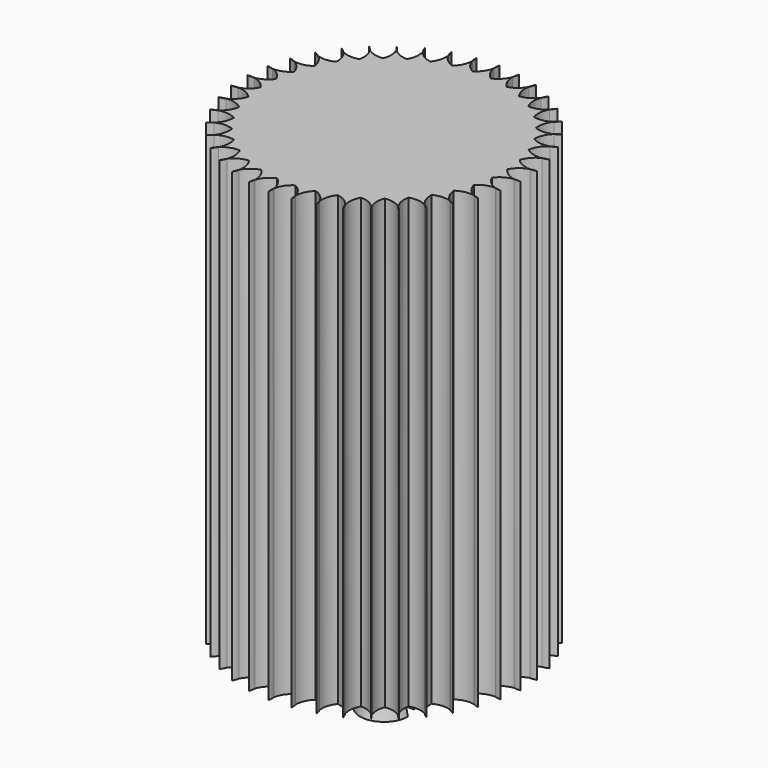
from build123d import *

# Parameters (mm, degrees)
F1_DEPTH  = 76.2
F2_R      = 43.4133239612
F3_DEPTH  = 101.6
F4_R      = 43.4133239612
F4_R_2    = 37.0604251076
F5_DEPTH  = 25.4
F5_TAPER  = -12
F6_W      = 117.5021827221
F6_H      = 89.2960429192
F7_DEPTH  = 25.4
F9_DEPTH  = 914.4
F11_R     = 53.1430060109
F11_R_2   = 54.2538976406
F12_DEPTH = 508


with BuildPart() as f1:
    # F0 (on Top) → F1 (new body)
    with BuildSketch(Plane.XY):
        with BuildLine():
            ThreePointArc((12.3147964478, 55.8442249894), (-0.0568873663, 74.6383593827), (-16.0615742207, 58.8229224086))
            Line((-16.0615742207, 58.8229224086), (-35.8245223761, 38.4155064821))
            Line((-35.8245223761, 38.4155064821), (-86.3886475563, 38.4155064821))
            Line((-86.3886475563, 38.4155064821), (-86.3886475563, -48.9976257086))
            Line((-86.3886475563, -48.9976257086), (99.40969944, -48.9976257086))
            Line((99.40969944, -48.9976257086), (101.6570031643, 38.4155064821))
            Line((101.6570031643, 38.4155064821), (32.9162478447, 38.4155064821))
            Line((32.9162478447, 38.4155064821), (12.3147964478, 55.8442249894))
        make_face()
    extrude(amount=F1_DEPTH)


with BuildPart() as f3:
    # F2 (on Top) → F3 (new body)
    with BuildSketch(Plane.XY):
        Circle(F2_R)
    extrude(amount=-F3_DEPTH)

    # F4 (on face) → F5 (join)
    with BuildSketch(Plane(origin=(0, 0, -101.6), x_dir=(1, 0, 0), z_dir=(0, 0, -1))):
        Circle(F4_R)
        Circle(F4_R_2, mode=Mode.SUBTRACT)
    extrude(amount=F5_DEPTH, taper=F5_TAPER)

    # F6 (on Front) → F7 (cut)
    with BuildSketch(Plane.XZ):
        with Locations((0, -93.4350788593)):
            Rectangle(F6_W, F6_H)
    extrude(amount=-F7_DEPTH, mode=Mode.SUBTRACT)


with BuildPart() as f9:
    # F8 (on Top) → F9 (new body)
    with BuildSketch(Plane.XY):
        with BuildLine():
            ThreePointArc((35.2223104144, -269.369402679), (35.5915835041, -275.9196411281), (36.9189268773, -282.3446038458))
            ThreePointArc((36.9189268773, -282.3446038458), (36.5496537876, -275.7943653967), (35.2223104144, -269.369402679))
        make_face()
    extrude(amount=F9_DEPTH)


with BuildPart() as f9b:
    # F8 (on Top) → F9, piece 2 (new body)
    with BuildSketch(Plane.XY):
        with BuildLine():
            ThreePointArc((-7.7040334356, -284.6438658243), (-7.0440771132, -278.1165046418), (-7.3499930812, -271.5630016263))
            ThreePointArc((-7.3499930812, -271.5630016263), (-8.0099494037, -278.0903628088), (-7.7040334356, -284.6438658243))
        make_face()
    extrude(amount=F9_DEPTH)


with BuildPart() as f9c:
    # F8 (on Top) → F9, piece 3 (new body)
    with BuildSketch(Plane.XY):
        with BuildLine():
            ThreePointArc((-52.1372948771, -279.9342511475), (-50.4643594574, -273.5904925269), (-49.7413153539, -267.0698182076))
            ThreePointArc((-49.7413153539, -267.0698182076), (-51.4142507736, -273.4135768282), (-52.1372948771, -279.9342511475))
        make_face()
    extrude(amount=F9_DEPTH)


with BuildPart() as f9d:
    # F8 (on Top) → F9, piece 4 (new body)
    with BuildSketch(Plane.XY):
        with BuildLine():
            ThreePointArc((-95.286763085, -268.3317261588), (-92.6420417903, -262.3277744912), (-90.9078413606, -256.0004895108))
            ThreePointArc((-90.9078413606, -256.0004895108), (-93.5525626554, -262.0044411784), (-95.286763085, -268.3317261588))
        make_face()
    extrude(amount=F9_DEPTH)


with BuildPart() as f9e:
    # F8 (on Top) → F9, piece 5 (new body)
    with BuildSketch(Plane.XY):
        with BuildLine():
            ThreePointArc((-136.0899549471, -250.1219835302), (-132.5385695929, -244.6056760315), (-129.8359146072, -238.6275791452))
            ThreePointArc((-129.8359146072, -238.6275791452), (-133.3872999614, -244.1438866439), (-136.0899549471, -250.1219835302))
        make_face()
    extrude(amount=F9_DEPTH)


with BuildPart() as f9f:
    # F8 (on Top) → F9, piece 6 (new body)
    with BuildSketch(Plane.XY):
        with BuildLine():
            ThreePointArc((-173.5421604617, -225.7534075598), (-169.1715579419, -220.8605740283), (-165.5669967354, -215.3788658216))
            ThreePointArc((-165.5669967354, -215.3788658216), (-169.9375992553, -220.2716993531), (-173.5421604617, -225.7534075598))
        make_face()
    extrude(amount=F9_DEPTH)


with BuildPart() as f9g:
    # F8 (on Top) → F9, piece 7 (new body)
    with BuildSketch(Plane.XY):
        with BuildLine():
            ThreePointArc((-206.7211820324, -195.8260334627), (-201.6389810861, -191.6771516982), (-197.2212699187, -186.82681002))
            ThreePointArc((-197.2212699187, -186.82681002), (-202.303470865, -190.9756917844), (-206.7211820324, -195.8260334627))
        make_face()
    extrude(amount=F9_DEPTH)


with BuildPart() as f9h:
    # F8 (on Top) → F9, piece 8 (new body)
    with BuildSketch(Plane.XY):
        with BuildLine():
            ThreePointArc((-234.8100420331, -161.0767725124), (-229.1413833145, -157.7740017534), (-224.0193008967, -153.674458113))
            ThreePointArc((-224.0193008967, -153.674458113), (-229.6879596153, -156.977228872), (-234.8100420331, -161.0767725124))
        make_face()
    extrude(amount=F9_DEPTH)


with BuildPart() as f9i:
    # F8 (on Top) → F9, piece 9 (new body)
    with BuildSketch(Plane.XY):
        with BuildLine():
            ThreePointArc((-257.1170995091, -122.3612668397), (-251.0015642092, -119.9859322634), (-245.3012332092, -116.738131031))
            ThreePointArc((-245.3012332092, -116.738131031), (-251.4167685092, -119.1134656072), (-257.1170995091, -122.3612668397))
        make_face()
    extrude(amount=F9_DEPTH)


with BuildPart() as f9j:
    # F8 (on Top) → F9, piece 10 (new body)
    with BuildSketch(Plane.XY):
        with BuildLine():
            ThreePointArc((-273.0930806725, -80.6328206836), (-266.6812535665, -79.2434109107), (-260.543035052, -76.9273237314))
            ThreePointArc((-260.543035052, -76.9273237314), (-266.954862158, -78.3167335043), (-273.0930806725, -80.6328206836))
        make_face()
    extrude(amount=F9_DEPTH)


with BuildPart() as f9k:
    # F8 (on Top) → F9, piece 11 (new body)
    with BuildSketch(Plane.XY):
        with BuildLine():
            ThreePointArc((-282.3446038458, -36.9189268773), (-275.7943653967, -36.5496537876), (-269.369402679, -35.2223104144))
            ThreePointArc((-269.369402679, -35.2223104144), (-275.9196411281, -35.5915835041), (-282.3446038458, -36.9189268773))
        make_face()
    extrude(amount=F9_DEPTH)


with BuildPart() as f9l:
    # F8 (on Top) → F9, piece 12 (new body)
    with BuildSketch(Plane.XY):
        with BuildLine():
            ThreePointArc((-284.6438658243, 7.7040334356), (-278.1165046418, 7.0440771132), (-271.5630016263, 7.3499930812))
            ThreePointArc((-271.5630016263, 7.3499930812), (-278.0903628088, 8.0099494037), (-284.6438658243, 7.7040334356))
        make_face()
    extrude(amount=F9_DEPTH)


with BuildPart() as f9m:
    # F8 (on Top) → F9, piece 13 (new body)
    with BuildSketch(Plane.XY):
        with BuildLine():
            ThreePointArc((-279.9342511475, 52.1372948771), (-273.5904925269, 50.4643594574), (-267.0698182076, 49.7413153539))
            ThreePointArc((-267.0698182076, 49.7413153539), (-273.4135768282, 51.4142507736), (-279.9342511475, 52.1372948771))
        make_face()
    extrude(amount=F9_DEPTH)


with BuildPart() as f9n:
    # F8 (on Top) → F9, piece 14 (new body)
    with BuildSketch(Plane.XY):
        with BuildLine():
            ThreePointArc((-268.3317261588, 95.286763085), (-262.3277744912, 92.6420417903), (-256.0004895108, 90.9078413606))
            ThreePointArc((-256.0004895108, 90.9078413606), (-262.0044411784, 93.5525626554), (-268.3317261588, 95.286763085))
        make_face()
    extrude(amount=F9_DEPTH)


with BuildPart() as f9o:
    # F8 (on Top) → F9, piece 15 (new body)
    with BuildSketch(Plane.XY):
        with BuildLine():
            ThreePointArc((-250.1219835302, 136.0899549471), (-244.6056760315, 132.5385695929), (-238.6275791452, 129.8359146072))
            ThreePointArc((-238.6275791452, 129.8359146072), (-244.1438866439, 133.3872999614), (-250.1219835302, 136.0899549471))
        make_face()
    extrude(amount=F9_DEPTH)


with BuildPart() as f9p:
    # F8 (on Top) → F9, piece 16 (new body)
    with BuildSketch(Plane.XY):
        with BuildLine():
            ThreePointArc((-225.7534075598, 173.5421604617), (-220.8605740283, 169.1715579419), (-215.3788658216, 165.5669967354))
            ThreePointArc((-215.3788658216, 165.5669967354), (-220.2716993531, 169.9375992553), (-225.7534075598, 173.5421604617))
        make_face()
    extrude(amount=F9_DEPTH)


with BuildPart() as f9q:
    # F8 (on Top) → F9, piece 17 (new body)
    with BuildSketch(Plane.XY):
        with BuildLine():
            ThreePointArc((-195.8260334627, 206.7211820324), (-191.6771516982, 201.6389810861), (-186.82681002, 197.2212699187))
            ThreePointArc((-186.82681002, 197.2212699187), (-190.9756917844, 202.303470865), (-195.8260334627, 206.7211820324))
        make_face()
    extrude(amount=F9_DEPTH)


with BuildPart() as f9r:
    # F8 (on Top) → F9, piece 18 (new body)
    with BuildSketch(Plane.XY):
        with BuildLine():
            ThreePointArc((-161.0767725124, 234.8100420331), (-157.7740017534, 229.1413833145), (-153.674458113, 224.0193008967))
            ThreePointArc((-153.674458113, 224.0193008967), (-156.977228872, 229.6879596153), (-161.0767725124, 234.8100420331))
        make_face()
    extrude(amount=F9_DEPTH)


with BuildPart() as f9s:
    # F8 (on Top) → F9, piece 19 (new body)
    with BuildSketch(Plane.XY):
        with BuildLine():
            ThreePointArc((-122.3612668397, 257.1170995091), (-119.9859322634, 251.0015642092), (-116.738131031, 245.3012332092))
            ThreePointArc((-116.738131031, 245.3012332092), (-119.1134656072, 251.4167685092), (-122.3612668397, 257.1170995091))
        make_face()
    extrude(amount=F9_DEPTH)


with BuildPart() as f9t:
    # F8 (on Top) → F9, piece 20 (new body)
    with BuildSketch(Plane.XY):
        with BuildLine():
            ThreePointArc((-80.6328206836, 273.0930806725), (-79.2434109107, 266.6812535665), (-76.9273237314, 260.543035052))
            ThreePointArc((-76.9273237314, 260.543035052), (-78.3167335043, 266.954862158), (-80.6328206836, 273.0930806725))
        make_face()
    extrude(amount=F9_DEPTH)


with BuildPart() as f9u:
    # F8 (on Top) → F9, piece 21 (new body)
    with BuildSketch(Plane.XY):
        with BuildLine():
            ThreePointArc((-36.9189268773, 282.3446038458), (-36.5496537876, 275.7943653967), (-35.2223104144, 269.369402679))
            ThreePointArc((-35.2223104144, 269.369402679), (-35.5915835041, 275.9196411281), (-36.9189268773, 282.3446038458))
        make_face()
    extrude(amount=F9_DEPTH)


with BuildPart() as f9v:
    # F8 (on Top) → F9, piece 22 (new body)
    with BuildSketch(Plane.XY):
        with BuildLine():
            ThreePointArc((7.7040334356, 284.6438658243), (7.0440771132, 278.1165046418), (7.3499930812, 271.5630016263))
            ThreePointArc((7.3499930812, 271.5630016263), (8.0099494037, 278.0903628088), (7.7040334356, 284.6438658243))
        make_face()
    extrude(amount=F9_DEPTH)


with BuildPart() as f9w:
    # F8 (on Top) → F9, piece 23 (new body)
    with BuildSketch(Plane.XY):
        with BuildLine():
            ThreePointArc((52.1372948771, 279.9342511475), (50.4643594574, 273.5904925269), (49.7413153539, 267.0698182076))
            ThreePointArc((49.7413153539, 267.0698182076), (51.4142507736, 273.4135768282), (52.1372948771, 279.9342511475))
        make_face()
    extrude(amount=F9_DEPTH)


with BuildPart() as f9x:
    # F8 (on Top) → F9, piece 24 (new body)
    with BuildSketch(Plane.XY):
        with BuildLine():
            ThreePointArc((95.286763085, 268.3317261588), (92.6420417903, 262.3277744912), (90.9078413606, 256.0004895108))
            ThreePointArc((90.9078413606, 256.0004895108), (93.5525626554, 262.0044411784), (95.286763085, 268.3317261588))
        make_face()
    extrude(amount=F9_DEPTH)


with BuildPart() as f9y:
    # F8 (on Top) → F9, piece 25 (new body)
    with BuildSketch(Plane.XY):
        with BuildLine():
            ThreePointArc((136.0899549471, 250.1219835302), (132.5385695929, 244.6056760315), (129.8359146072, 238.6275791452))
            ThreePointArc((129.8359146072, 238.6275791452), (133.3872999614, 244.1438866439), (136.0899549471, 250.1219835302))
        make_face()
    extrude(amount=F9_DEPTH)


with BuildPart() as f9z:
    # F8 (on Top) → F9, piece 26 (new body)
    with BuildSketch(Plane.XY):
        with BuildLine():
            ThreePointArc((173.5421604617, 225.7534075598), (169.1715579419, 220.8605740283), (165.5669967354, 215.3788658216))
            ThreePointArc((165.5669967354, 215.3788658216), (169.9375992553, 220.2716993531), (173.5421604617, 225.7534075598))
        make_face()
    extrude(amount=F9_DEPTH)


with BuildPart() as f9ba:
    # F8 (on Top) → F9, piece 27 (new body)
    with BuildSketch(Plane.XY):
        with BuildLine():
            ThreePointArc((206.7211820324, 195.8260334627), (201.6389810861, 191.6771516982), (197.2212699187, 186.82681002))
            ThreePointArc((197.2212699187, 186.82681002), (202.303470865, 190.9756917844), (206.7211820324, 195.8260334627))
        make_face()
    extrude(amount=F9_DEPTH)


with BuildPart() as f9bb:
    # F8 (on Top) → F9, piece 28 (new body)
    with BuildSketch(Plane.XY):
        with BuildLine():
            ThreePointArc((234.8100420331, 161.0767725124), (229.1413833145, 157.7740017534), (224.0193008967, 153.674458113))
            ThreePointArc((224.0193008967, 153.674458113), (229.6879596153, 156.977228872), (234.8100420331, 161.0767725124))
        make_face()
    extrude(amount=F9_DEPTH)


with BuildPart() as f9bc:
    # F8 (on Top) → F9, piece 29 (new body)
    with BuildSketch(Plane.XY):
        with BuildLine():
            ThreePointArc((257.1170995091, 122.3612668397), (251.0015642092, 119.9859322634), (245.3012332092, 116.738131031))
            ThreePointArc((245.3012332092, 116.738131031), (251.4167685092, 119.1134656072), (257.1170995091, 122.3612668397))
        make_face()
    extrude(amount=F9_DEPTH)


with BuildPart() as f9bd:
    # F8 (on Top) → F9, piece 30 (new body)
    with BuildSketch(Plane.XY):
        with BuildLine():
            ThreePointArc((273.0930806725, 80.6328206836), (266.6812535665, 79.2434109107), (260.543035052, 76.9273237314))
            ThreePointArc((260.543035052, 76.9273237314), (266.954862158, 78.3167335043), (273.0930806725, 80.6328206836))
        make_face()
    extrude(amount=F9_DEPTH)


with BuildPart() as f9be:
    # F8 (on Top) → F9, piece 31 (new body)
    with BuildSketch(Plane.XY):
        with BuildLine():
            ThreePointArc((282.3446038458, 36.9189268773), (275.7943653967, 36.5496537876), (269.369402679, 35.2223104144))
            ThreePointArc((269.369402679, 35.2223104144), (275.9196411281, 35.5915835041), (282.3446038458, 36.9189268773))
        make_face()
    extrude(amount=F9_DEPTH)


with BuildPart() as f9bf:
    # F8 (on Top) → F9, piece 32 (new body)
    with BuildSketch(Plane.XY):
        with BuildLine():
            ThreePointArc((284.6438658243, -7.7040334356), (278.1165046418, -7.0440771132), (271.5630016263, -7.3499930812))
            ThreePointArc((271.5630016263, -7.3499930812), (278.0903628088, -8.0099494037), (284.6438658243, -7.7040334356))
        make_face()
    extrude(amount=F9_DEPTH)


with BuildPart() as f9bg:
    # F8 (on Top) → F9, piece 33 (new body)
    with BuildSketch(Plane.XY):
        with BuildLine():
            ThreePointArc((279.9342511475, -52.1372948771), (273.5904925269, -50.4643594574), (267.0698182076, -49.7413153539))
            ThreePointArc((267.0698182076, -49.7413153539), (273.4135768282, -51.4142507736), (279.9342511475, -52.1372948771))
        make_face()
    extrude(amount=F9_DEPTH)


with BuildPart() as f9bh:
    # F8 (on Top) → F9, piece 34 (new body)
    with BuildSketch(Plane.XY):
        with BuildLine():
            ThreePointArc((268.3317261588, -95.286763085), (262.3277744912, -92.6420417903), (256.0004895108, -90.9078413606))
            ThreePointArc((256.0004895108, -90.9078413606), (262.0044411784, -93.5525626554), (268.3317261588, -95.286763085))
        make_face()
    extrude(amount=F9_DEPTH)


with BuildPart() as f9bi:
    # F8 (on Top) → F9, piece 35 (new body)
    with BuildSketch(Plane.XY):
        with BuildLine():
            ThreePointArc((250.1219835302, -136.0899549471), (244.6056760315, -132.5385695929), (238.6275791452, -129.8359146072))
            ThreePointArc((238.6275791452, -129.8359146072), (244.1438866439, -133.3872999614), (250.1219835302, -136.0899549471))
        make_face()
    extrude(amount=F9_DEPTH)


with BuildPart() as f9bj:
    # F8 (on Top) → F9, piece 36 (new body)
    with BuildSketch(Plane.XY):
        with BuildLine():
            ThreePointArc((225.7534075598, -173.5421604617), (220.8605740283, -169.1715579419), (215.3788658216, -165.5669967354))
            ThreePointArc((215.3788658216, -165.5669967354), (220.2716993531, -169.9375992553), (225.7534075598, -173.5421604617))
        make_face()
    extrude(amount=F9_DEPTH)


with BuildPart() as f9bk:
    # F8 (on Top) → F9, piece 37 (new body)
    with BuildSketch(Plane.XY):
        with BuildLine():
            ThreePointArc((195.8260334627, -206.7211820324), (191.6771516982, -201.6389810861), (186.82681002, -197.2212699187))
            ThreePointArc((186.82681002, -197.2212699187), (190.9756917844, -202.303470865), (195.8260334627, -206.7211820324))
        make_face()
    extrude(amount=F9_DEPTH)


with BuildPart() as f9bl:
    # F8 (on Top) → F9, piece 38 (new body)
    with BuildSketch(Plane.XY):
        with BuildLine():
            ThreePointArc((161.0767725124, -234.8100420331), (157.7740017534, -229.1413833145), (153.674458113, -224.0193008967))
            ThreePointArc((153.674458113, -224.0193008967), (156.977228872, -229.6879596153), (161.0767725124, -234.8100420331))
        make_face()
    extrude(amount=F9_DEPTH)


with BuildPart() as f9bm:
    # F8 (on Top) → F9, piece 39 (new body)
    with BuildSketch(Plane.XY):
        with BuildLine():
            ThreePointArc((122.3612668397, -257.1170995091), (119.9859322634, -251.0015642092), (116.738131031, -245.3012332092))
            ThreePointArc((116.738131031, -245.3012332092), (119.1134656072, -251.4167685092), (122.3612668397, -257.1170995091))
        make_face()
    extrude(amount=F9_DEPTH)


with BuildPart() as f9bn:
    # F8 (on Top) → F9, piece 40 (new body)
    with BuildSketch(Plane.XY):
        with BuildLine():
            ThreePointArc((80.6328206836, -273.0930806725), (79.2434109107, -266.6812535665), (76.9273237314, -260.543035052))
            ThreePointArc((76.9273237314, -260.543035052), (78.3167335043, -266.954862158), (80.6328206836, -273.0930806725))
        make_face()
    extrude(amount=F9_DEPTH)


with BuildPart() as f9bo:
    # F8 (on Top) → F9, piece 41 (new body)
    with BuildSketch(Plane.XY):
        with BuildLine():
            ThreePointArc((12.4594028501, -241.8060421514), (26.7269848942, -253.204244146), (35.2223104144, -269.369402679))
            ThreePointArc((35.2223104144, -269.369402679), (39.2756220508, -251.5634045079), (50.1328057733, -236.8799284988))
            ThreePointArc((50.1328057733, -236.8799284988), (30.7445808324, -235.1251032945), (12.4594028501, -241.8060421514))
        make_face()
        with BuildLine():
            ThreePointArc((-7.3499930812, -271.5630016263), (-0.5611126387, -254.6103024775), (12.4594028501, -241.8060421514))
            ThreePointArc((12.4594028501, -241.8060421514), (-6.4156057267, -237.0398351606), (-25.5207919216, -240.778088538))
            ThreePointArc((-25.5207919216, -240.778088538), (-13.2119391196, -254.2679013162), (-7.3499930812, -271.5630016263))
        make_face()
        with BuildLine():
            ThreePointArc((-25.5207919216, -240.778088538), (-6.4156057267, -237.0398351606), (12.4594028501, -241.8060421514))
            ThreePointArc((12.4594028501, -241.8060421514), (30.7445808324, -235.1251032945), (50.1328057733, -236.8799284988))
            ThreePointArc((50.1328057733, -236.8799284988), (67.1477337761, -227.4208110498), (86.5717726371, -226.1210448472))
            ThreePointArc((86.5717726371, -226.1210448472), (101.8974866636, -214.1166636707), (120.8790551433, -209.7943106187))
            ThreePointArc((120.8790551433, -209.7943106187), (134.1381852511, -195.5402534195), (152.2098941373, -188.3017441954))
            ThreePointArc((152.2098941373, -188.3017441954), (163.0759565386, -172.1489931682), (179.792820382, -162.1725638923))
            ThreePointArc((179.792820382, -162.1725638923), (187.9982565581, -144.5188533754), (202.9486506907, -132.0501568463))
            ThreePointArc((202.9486506907, -132.0501568463), (208.2914155706, -113.3301797819), (221.1072116715, -98.6762366894))
            ThreePointArc((221.1072116715, -98.6762366894), (223.4557486523, -79.3509410408), (233.8213792881, -62.8725800976))
            ThreePointArc((233.8213792881, -62.8725800976), (233.117859595, -43.4178187807), (240.778088538, -25.5207919216))
            ThreePointArc((240.778088538, -25.5207919216), (237.0398351606, -6.4156057267), (241.8060421514, 12.4594028501))
            ThreePointArc((241.8060421514, 12.4594028501), (235.1251032945, 30.7445808324), (236.8799284988, 50.1328057733))
            ThreePointArc((236.8799284988, 50.1328057733), (227.4208110498, 67.1477337761), (226.1210448472, 86.5717726371))
            ThreePointArc((226.1210448472, 86.5717726371), (214.1166636707, 101.8974866636), (209.7943106187, 120.8790551433))
            ThreePointArc((209.7943106187, 120.8790551433), (195.5402534195, 134.1381852511), (188.3017441954, 152.2098941373))
            ThreePointArc((188.3017441954, 152.2098941373), (172.1489931682, 163.0759565386), (162.1725638923, 179.792820382))
            ThreePointArc((162.1725638923, 179.792820382), (144.5188533754, 187.9982565581), (132.0501568463, 202.9486506907))
            ThreePointArc((132.0501568463, 202.9486506907), (113.3301797819, 208.2914155706), (98.6762366894, 221.1072116715))
            ThreePointArc((98.6762366894, 221.1072116715), (79.3509410408, 223.4557486523), (62.8725800976, 233.8213792881))
            ThreePointArc((62.8725800976, 233.8213792881), (43.4178187807, 233.117859595), (25.5207919216, 240.778088538))
            ThreePointArc((25.5207919216, 240.778088538), (6.4156057267, 237.0398351606), (-12.4594028501, 241.8060421514))
            ThreePointArc((-12.4594028501, 241.8060421514), (-30.7445808324, 235.1251032945), (-50.1328057733, 236.8799284988))
            ThreePointArc((-50.1328057733, 236.8799284988), (-67.1477337761, 227.4208110498), (-86.5717726371, 226.1210448472))
            ThreePointArc((-86.5717726371, 226.1210448472), (-101.8974866636, 214.1166636707), (-120.8790551433, 209.7943106187))
            ThreePointArc((-120.8790551433, 209.7943106187), (-134.1381852511, 195.5402534195), (-152.2098941373, 188.3017441954))
            ThreePointArc((-152.2098941373, 188.3017441954), (-163.0759565386, 172.1489931682), (-179.792820382, 162.1725638923))
            ThreePointArc((-179.792820382, 162.1725638923), (-187.9982565581, 144.5188533754), (-202.9486506907, 132.0501568463))
            ThreePointArc((-202.9486506907, 132.0501568463), (-208.2914155706, 113.3301797819), (-221.1072116715, 98.6762366894))
            ThreePointArc((-221.1072116715, 98.6762366894), (-223.4557486523, 79.3509410408), (-233.8213792881, 62.8725800976))
            ThreePointArc((-233.8213792881, 62.8725800976), (-233.117859595, 43.4178187807), (-240.778088538, 25.5207919216))
            ThreePointArc((-240.778088538, 25.5207919216), (-237.0398351606, 6.4156057267), (-241.8060421514, -12.4594028501))
            ThreePointArc((-241.8060421514, -12.4594028501), (-235.1251032945, -30.7445808324), (-236.8799284988, -50.1328057733))
            ThreePointArc((-236.8799284988, -50.1328057733), (-227.4208110498, -67.1477337761), (-226.1210448472, -86.5717726371))
            ThreePointArc((-226.1210448472, -86.5717726371), (-214.1166636707, -101.8974866636), (-209.7943106187, -120.8790551433))
            ThreePointArc((-209.7943106187, -120.8790551433), (-195.5402534195, -134.1381852511), (-188.3017441954, -152.2098941373))
            ThreePointArc((-188.3017441954, -152.2098941373), (-172.1489931682, -163.0759565386), (-162.1725638923, -179.792820382))
            ThreePointArc((-162.1725638923, -179.792820382), (-144.5188533754, -187.9982565581), (-132.0501568463, -202.9486506907))
            ThreePointArc((-132.0501568463, -202.9486506907), (-113.3301797819, -208.2914155706), (-98.6762366894, -221.1072116715))
            ThreePointArc((-98.6762366894, -221.1072116715), (-79.3509410408, -223.4557486523), (-62.8725800976, -233.8213792881))
            ThreePointArc((-62.8725800976, -233.8213792881), (-43.4178187807, -233.117859595), (-25.5207919216, -240.778088538))
        make_face()
        with BuildLine():
            ThreePointArc((86.5717726371, -226.1210448472), (67.1477337761, -227.4208110498), (50.1328057733, -236.8799284988))
            ThreePointArc((50.1328057733, -236.8799284988), (66.0078018382, -245.9058581481), (76.9273237314, -260.543035052))
            ThreePointArc((76.9273237314, -260.543035052), (78.1452605771, -242.3221806282), (86.5717726371, -226.1210448472))
        make_face()
        with BuildLine():
            ThreePointArc((-49.7413153539, -267.0698182076), (-40.3840308728, -251.3878497969), (-25.5207919216, -240.778088538))
            ThreePointArc((-25.5207919216, -240.778088538), (-43.4178187807, -233.117859595), (-62.8725800976, -233.8213792881))
            ThreePointArc((-62.8725800976, -233.8213792881), (-52.8255413444, -249.0706388893), (-49.7413153539, -267.0698182076))
        make_face()
        with BuildLine():
            ThreePointArc((120.8790551433, -209.7943106187), (101.8974866636, -214.1166636707), (86.5717726371, -226.1210448472))
            ThreePointArc((86.5717726371, -226.1210448472), (103.6632876335, -232.5524538079), (116.738131031, -245.3012332092))
            ThreePointArc((116.738131031, -245.3012332092), (115.0907034387, -227.1141804403), (120.8790551433, -209.7943106187))
        make_face()
        with BuildLine():
            ThreePointArc((-90.9078413606, -256.0004895108), (-79.2125602399, -241.975393946), (-62.8725800976, -233.8213792881))
            ThreePointArc((-62.8725800976, -233.8213792881), (-79.3509410408, -223.4557486523), (-98.6762366894, -221.1072116715))
            ThreePointArc((-98.6762366894, -221.1072116715), (-91.1384034234, -237.7404307149), (-90.9078413606, -256.0004895108))
        make_face()
        with BuildLine():
            ThreePointArc((152.2098941373, -188.3017441954), (134.1381852511, -195.5402534195), (120.8790551433, -209.7943106187))
            ThreePointArc((120.8790551433, -209.7943106187), (138.7662392486, -213.4728362576), (153.674458113, -224.0193008967))
            ThreePointArc((153.674458113, -224.0193008967), (149.2022312175, -206.3138753811), (152.2098941373, -188.3017441954))
        make_face()
        with BuildLine():
            ThreePointArc((-129.8359146072, -238.6275791452), (-116.0906134825, -226.6047008257), (-98.6762366894, -221.1072116715))
            ThreePointArc((-98.6762366894, -221.1072116715), (-113.3301797819, -208.2914155706), (-132.0501568463, -202.9486506907))
            ThreePointArc((-132.0501568463, -202.9486506907), (-127.2071355391, -220.556264121), (-129.8359146072, -238.6275791452))
        make_face()
        with BuildLine():
            ThreePointArc((179.792820382, -162.1725638923), (163.0759565386, -172.1489931682), (152.2098941373, -188.3017441954))
            ThreePointArc((152.2098941373, -188.3017441954), (170.4523055147, -189.1368090029), (186.82681002, -197.2212699187))
            ThreePointArc((186.82681002, -197.2212699187), (179.6399048899, -180.4334379936), (179.792820382, -162.1725638923))
        make_face()
        with BuildLine():
            ThreePointArc((-165.5669967354, -215.3788658216), (-150.1101305385, -205.6542479133), (-132.0501568463, -202.9486506907))
            ThreePointArc((-132.0501568463, -202.9486506907), (-144.5188533754, -187.9982565581), (-162.1725638923, -179.792820382))
            ThreePointArc((-162.1725638923, -179.792820382), (-160.1436058015, -197.9412703202), (-165.5669967354, -215.3788658216))
        make_face()
        with BuildLine():
            ThreePointArc((202.9486506907, -132.0501568463), (187.9982565581, -144.5188533754), (179.792820382, -162.1725638923))
            ThreePointArc((179.792820382, -162.1725638923), (197.9412703202, -160.1436058015), (215.3788658216, -165.5669967354))
            ThreePointArc((215.3788658216, -165.5669967354), (205.6542479133, -150.1101305385), (202.9486506907, -132.0501568463))
        make_face()
        with BuildLine():
            ThreePointArc((-197.2212699187, -186.82681002), (-180.4334379936, -179.6399048899), (-162.1725638923, -179.792820382))
            ThreePointArc((-162.1725638923, -179.792820382), (-172.1489931682, -163.0759565386), (-188.3017441954, -152.2098941373))
            ThreePointArc((-188.3017441954, -152.2098941373), (-189.1368090029, -170.4523055147), (-197.2212699187, -186.82681002))
        make_face()
        with BuildLine():
            ThreePointArc((221.1072116715, -98.6762366894), (208.2914155706, -113.3301797819), (202.9486506907, -132.0501568463))
            ThreePointArc((202.9486506907, -132.0501568463), (220.556264121, -127.2071355391), (238.6275791452, -129.8359146072))
            ThreePointArc((238.6275791452, -129.8359146072), (226.6047008257, -116.0906134825), (221.1072116715, -98.6762366894))
        make_face()
        with BuildLine():
            ThreePointArc((-224.0193008967, -153.674458113), (-206.3138753811, -149.2022312175), (-188.3017441954, -152.2098941373))
            ThreePointArc((-188.3017441954, -152.2098941373), (-195.5402534195, -134.1381852511), (-209.7943106187, -120.8790551433))
            ThreePointArc((-209.7943106187, -120.8790551433), (-213.4728362576, -138.7662392486), (-224.0193008967, -153.674458113))
        make_face()
        with BuildLine():
            ThreePointArc((233.8213792881, -62.8725800976), (223.4557486523, -79.3509410408), (221.1072116715, -98.6762366894))
            ThreePointArc((221.1072116715, -98.6762366894), (237.7404307149, -91.1384034234), (256.0004895108, -90.9078413606))
            ThreePointArc((256.0004895108, -90.9078413606), (241.975393946, -79.2125602399), (233.8213792881, -62.8725800976))
        make_face()
        with BuildLine():
            ThreePointArc((-245.3012332092, -116.738131031), (-227.1141804403, -115.0907034387), (-209.7943106187, -120.8790551433))
            ThreePointArc((-209.7943106187, -120.8790551433), (-214.1166636707, -101.8974866636), (-226.1210448472, -86.5717726371))
            ThreePointArc((-226.1210448472, -86.5717726371), (-232.5524538079, -103.6632876335), (-245.3012332092, -116.738131031))
        make_face()
        with BuildLine():
            ThreePointArc((240.778088538, -25.5207919216), (233.117859595, -43.4178187807), (233.8213792881, -62.8725800976))
            ThreePointArc((233.8213792881, -62.8725800976), (249.0706388893, -52.8255413444), (267.0698182076, -49.7413153539))
            ThreePointArc((267.0698182076, -49.7413153539), (251.3878497969, -40.3840308728), (240.778088538, -25.5207919216))
        make_face()
        with BuildLine():
            ThreePointArc((-260.543035052, -76.9273237314), (-242.3221806282, -78.1452605771), (-226.1210448472, -86.5717726371))
            ThreePointArc((-226.1210448472, -86.5717726371), (-227.4208110498, -67.1477337761), (-236.8799284988, -50.1328057733))
            ThreePointArc((-236.8799284988, -50.1328057733), (-245.9058581481, -66.0078018382), (-260.543035052, -76.9273237314))
        make_face()
        with BuildLine():
            ThreePointArc((241.8060421514, 12.4594028501), (237.0398351606, -6.4156057267), (240.778088538, -25.5207919216))
            ThreePointArc((240.778088538, -25.5207919216), (254.2679013162, -13.2119391196), (271.5630016263, -7.3499930812))
            ThreePointArc((271.5630016263, -7.3499930812), (254.6103024775, -0.5611126387), (241.8060421514, 12.4594028501))
        make_face()
        with BuildLine():
            ThreePointArc((-269.369402679, -35.2223104144), (-251.5634045079, -39.2756220508), (-236.8799284988, -50.1328057733))
            ThreePointArc((-236.8799284988, -50.1328057733), (-235.1251032945, -30.7445808324), (-241.8060421514, -12.4594028501))
            ThreePointArc((-241.8060421514, -12.4594028501), (-253.204244146, -26.7269848942), (-269.369402679, -35.2223104144))
        make_face()
        with BuildLine():
            ThreePointArc((236.8799284988, 50.1328057733), (235.1251032945, 30.7445808324), (241.8060421514, 12.4594028501))
            ThreePointArc((241.8060421514, 12.4594028501), (253.204244146, 26.7269848942), (269.369402679, 35.2223104144))
            ThreePointArc((269.369402679, 35.2223104144), (251.5634045079, 39.2756220508), (236.8799284988, 50.1328057733))
        make_face()
        with BuildLine():
            ThreePointArc((-271.5630016263, 7.3499930812), (-254.6103024775, 0.5611126387), (-241.8060421514, -12.4594028501))
            ThreePointArc((-241.8060421514, -12.4594028501), (-237.0398351606, 6.4156057267), (-240.778088538, 25.5207919216))
            ThreePointArc((-240.778088538, 25.5207919216), (-254.2679013162, 13.2119391196), (-271.5630016263, 7.3499930812))
        make_face()
        with BuildLine():
            ThreePointArc((226.1210448472, 86.5717726371), (227.4208110498, 67.1477337761), (236.8799284988, 50.1328057733))
            ThreePointArc((236.8799284988, 50.1328057733), (245.9058581481, 66.0078018382), (260.543035052, 76.9273237314))
            ThreePointArc((260.543035052, 76.9273237314), (242.3221806282, 78.1452605771), (226.1210448472, 86.5717726371))
        make_face()
        with BuildLine():
            ThreePointArc((-267.0698182076, 49.7413153539), (-251.3878497969, 40.3840308728), (-240.778088538, 25.5207919216))
            ThreePointArc((-240.778088538, 25.5207919216), (-233.117859595, 43.4178187807), (-233.8213792881, 62.8725800976))
            ThreePointArc((-233.8213792881, 62.8725800976), (-249.0706388893, 52.8255413444), (-267.0698182076, 49.7413153539))
        make_face()
        with BuildLine():
            ThreePointArc((209.7943106187, 120.8790551433), (214.1166636707, 101.8974866636), (226.1210448472, 86.5717726371))
            ThreePointArc((226.1210448472, 86.5717726371), (232.5524538079, 103.6632876335), (245.3012332092, 116.738131031))
            ThreePointArc((245.3012332092, 116.738131031), (227.1141804403, 115.0907034387), (209.7943106187, 120.8790551433))
        make_face()
        with BuildLine():
            ThreePointArc((-256.0004895108, 90.9078413606), (-241.975393946, 79.2125602399), (-233.8213792881, 62.8725800976))
            ThreePointArc((-233.8213792881, 62.8725800976), (-223.4557486523, 79.3509410408), (-221.1072116715, 98.6762366894))
            ThreePointArc((-221.1072116715, 98.6762366894), (-237.7404307149, 91.1384034234), (-256.0004895108, 90.9078413606))
        make_face()
        with BuildLine():
            ThreePointArc((188.3017441954, 152.2098941373), (195.5402534195, 134.1381852511), (209.7943106187, 120.8790551433))
            ThreePointArc((209.7943106187, 120.8790551433), (213.4728362576, 138.7662392486), (224.0193008967, 153.674458113))
            ThreePointArc((224.0193008967, 153.674458113), (206.3138753811, 149.2022312175), (188.3017441954, 152.2098941373))
        make_face()
        with BuildLine():
            ThreePointArc((-238.6275791452, 129.8359146072), (-226.6047008257, 116.0906134825), (-221.1072116715, 98.6762366894))
            ThreePointArc((-221.1072116715, 98.6762366894), (-208.2914155706, 113.3301797819), (-202.9486506907, 132.0501568463))
            ThreePointArc((-202.9486506907, 132.0501568463), (-220.556264121, 127.2071355391), (-238.6275791452, 129.8359146072))
        make_face()
        with BuildLine():
            ThreePointArc((162.1725638923, 179.792820382), (172.1489931682, 163.0759565386), (188.3017441954, 152.2098941373))
            ThreePointArc((188.3017441954, 152.2098941373), (189.1368090029, 170.4523055147), (197.2212699187, 186.82681002))
            ThreePointArc((197.2212699187, 186.82681002), (180.4334379936, 179.6399048899), (162.1725638923, 179.792820382))
        make_face()
        with BuildLine():
            ThreePointArc((-215.3788658216, 165.5669967354), (-205.6542479133, 150.1101305385), (-202.9486506907, 132.0501568463))
            ThreePointArc((-202.9486506907, 132.0501568463), (-187.9982565581, 144.5188533754), (-179.792820382, 162.1725638923))
            ThreePointArc((-179.792820382, 162.1725638923), (-197.9412703202, 160.1436058015), (-215.3788658216, 165.5669967354))
        make_face()
        with BuildLine():
            ThreePointArc((132.0501568463, 202.9486506907), (144.5188533754, 187.9982565581), (162.1725638923, 179.792820382))
            ThreePointArc((162.1725638923, 179.792820382), (160.1436058015, 197.9412703202), (165.5669967354, 215.3788658216))
            ThreePointArc((165.5669967354, 215.3788658216), (150.1101305385, 205.6542479133), (132.0501568463, 202.9486506907))
        make_face()
        with BuildLine():
            ThreePointArc((-186.82681002, 197.2212699187), (-179.6399048899, 180.4334379936), (-179.792820382, 162.1725638923))
            ThreePointArc((-179.792820382, 162.1725638923), (-163.0759565386, 172.1489931682), (-152.2098941373, 188.3017441954))
            ThreePointArc((-152.2098941373, 188.3017441954), (-170.4523055147, 189.1368090029), (-186.82681002, 197.2212699187))
        make_face()
        with BuildLine():
            ThreePointArc((98.6762366894, 221.1072116715), (113.3301797819, 208.2914155706), (132.0501568463, 202.9486506907))
            ThreePointArc((132.0501568463, 202.9486506907), (127.2071355391, 220.556264121), (129.8359146072, 238.6275791452))
            ThreePointArc((129.8359146072, 238.6275791452), (116.0906134825, 226.6047008257), (98.6762366894, 221.1072116715))
        make_face()
        with BuildLine():
            ThreePointArc((-153.674458113, 224.0193008967), (-149.2022312175, 206.3138753811), (-152.2098941373, 188.3017441954))
            ThreePointArc((-152.2098941373, 188.3017441954), (-134.1381852511, 195.5402534195), (-120.8790551433, 209.7943106187))
            ThreePointArc((-120.8790551433, 209.7943106187), (-138.7662392486, 213.4728362576), (-153.674458113, 224.0193008967))
        make_face()
        with BuildLine():
            ThreePointArc((62.8725800976, 233.8213792881), (79.3509410408, 223.4557486523), (98.6762366894, 221.1072116715))
            ThreePointArc((98.6762366894, 221.1072116715), (91.1384034234, 237.7404307149), (90.9078413606, 256.0004895108))
            ThreePointArc((90.9078413606, 256.0004895108), (79.2125602399, 241.975393946), (62.8725800976, 233.8213792881))
        make_face()
        with BuildLine():
            ThreePointArc((-116.738131031, 245.3012332092), (-115.0907034387, 227.1141804403), (-120.8790551433, 209.7943106187))
            ThreePointArc((-120.8790551433, 209.7943106187), (-101.8974866636, 214.1166636707), (-86.5717726371, 226.1210448472))
            ThreePointArc((-86.5717726371, 226.1210448472), (-103.6632876335, 232.5524538079), (-116.738131031, 245.3012332092))
        make_face()
        with BuildLine():
            ThreePointArc((25.5207919216, 240.778088538), (43.4178187807, 233.117859595), (62.8725800976, 233.8213792881))
            ThreePointArc((62.8725800976, 233.8213792881), (52.8255413444, 249.0706388893), (49.7413153539, 267.0698182076))
            ThreePointArc((49.7413153539, 267.0698182076), (40.3840308728, 251.3878497969), (25.5207919216, 240.778088538))
        make_face()
        with BuildLine():
            ThreePointArc((-76.9273237314, 260.543035052), (-78.1452605771, 242.3221806282), (-86.5717726371, 226.1210448472))
            ThreePointArc((-86.5717726371, 226.1210448472), (-67.1477337761, 227.4208110498), (-50.1328057733, 236.8799284988))
            ThreePointArc((-50.1328057733, 236.8799284988), (-66.0078018382, 245.9058581481), (-76.9273237314, 260.543035052))
        make_face()
        with BuildLine():
            ThreePointArc((-12.4594028501, 241.8060421514), (6.4156057267, 237.0398351606), (25.5207919216, 240.778088538))
            ThreePointArc((25.5207919216, 240.778088538), (13.2119391196, 254.2679013162), (7.3499930812, 271.5630016263))
            ThreePointArc((7.3499930812, 271.5630016263), (0.5611126387, 254.6103024775), (-12.4594028501, 241.8060421514))
        make_face()
        with BuildLine():
            ThreePointArc((-35.2223104144, 269.369402679), (-39.2756220508, 251.5634045079), (-50.1328057733, 236.8799284988))
            ThreePointArc((-50.1328057733, 236.8799284988), (-30.7445808324, 235.1251032945), (-12.4594028501, 241.8060421514))
            ThreePointArc((-12.4594028501, 241.8060421514), (-26.7269848942, 253.204244146), (-35.2223104144, 269.369402679))
        make_face()
    extrude(amount=F9_DEPTH)

    # F11 (on offset) → F12 (cut)
    with BuildSketch(Plane.XY.offset(381)):
        with Locations((123.2672780752, 0)):
            Circle(F11_R)
        with Locations((-126.4261752367, 0)):
            Circle(F11_R_2)
    extrude(amount=-F12_DEPTH, mode=Mode.SUBTRACT)


solid = Compound([f1.part, f3.part, f9.part, f9b.part, f9c.part, f9d.part, f9e.part, f9f.part, f9g.part, f9h.part, f9i.part, f9j.part, f9k.part, f9l.part, f9m.part, f9n.part, f9o.part, f9p.part, f9q.part, f9r.part, f9s.part, f9t.part, f9u.part, f9v.part, f9w.part, f9x.part, f9y.part, f9z.part, f9ba.part, f9bb.part, f9bc.part, f9bd.part, f9be.part, f9bf.part, f9bg.part, f9bh.part, f9bi.part, f9bj.part, f9bk.part, f9bl.part, f9bm.part, f9bn.part, f9bo.part])
